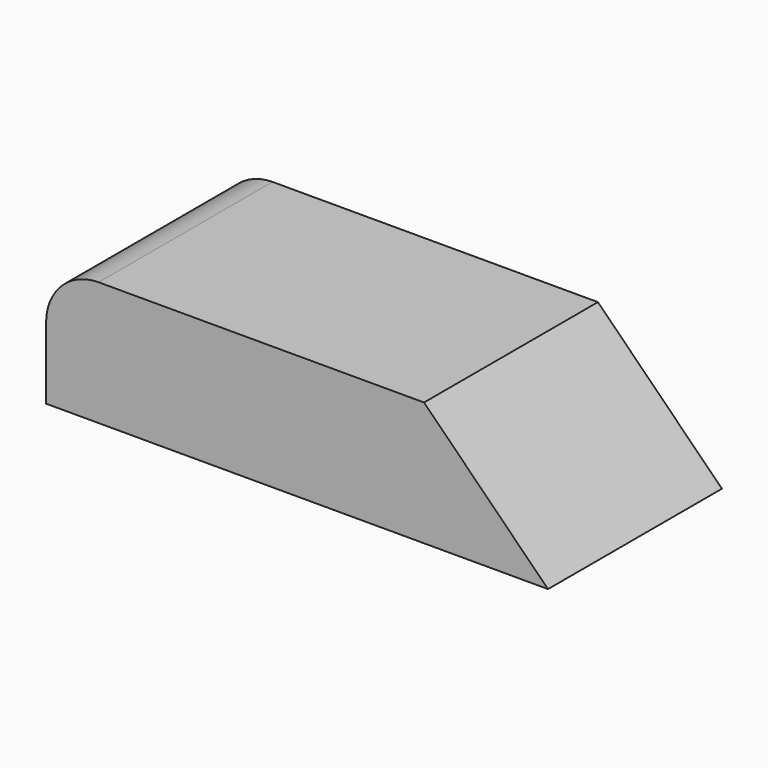
from build123d import *

# Parameters (mm, degrees)
F0_W        = 599.3404984474
F0_H        = 229.6551764011
F1_DEPTH    = 131
F2_R        = 55.5269119346
F3_T1_DEPTH = 1258.3283715875


# Not quite as in the source:
# - a fillet or chamfer that OpenCascade refuses, or shapes differently, is made with other operations: its cross-section is extruded or revolved along the edge and cut away or added


with BuildPart() as f1:
    # F0 (on Top) → F1 (new body)
    with BuildSketch(Plane.XY):
        with Locations((-30.9103131294, -57.0044666529)):
            Rectangle(F0_W, F0_H)
    extrude(amount=F1_DEPTH)

    # F2
    f2_edges = [f1.edges().sort_by_distance(p)[0] for p in [
        (-330.580562, -57.004467, 131),
    ]]
    fillet(f2_edges, radius=F2_R)

    # F3: chamfer of 200 on 1 edges, made by hand

    # F3_s2 → F3_t1 (cut)
    with BuildSketch(Plane.XZ.offset(-572.1597191409)):
        Polygon((68.7599360943, 131), (268.7599360943, -69), (268.7599360943, 131), align=None)
    extrude(amount=F3_T1_DEPTH, mode=Mode.SUBTRACT)


solid = f1.part
